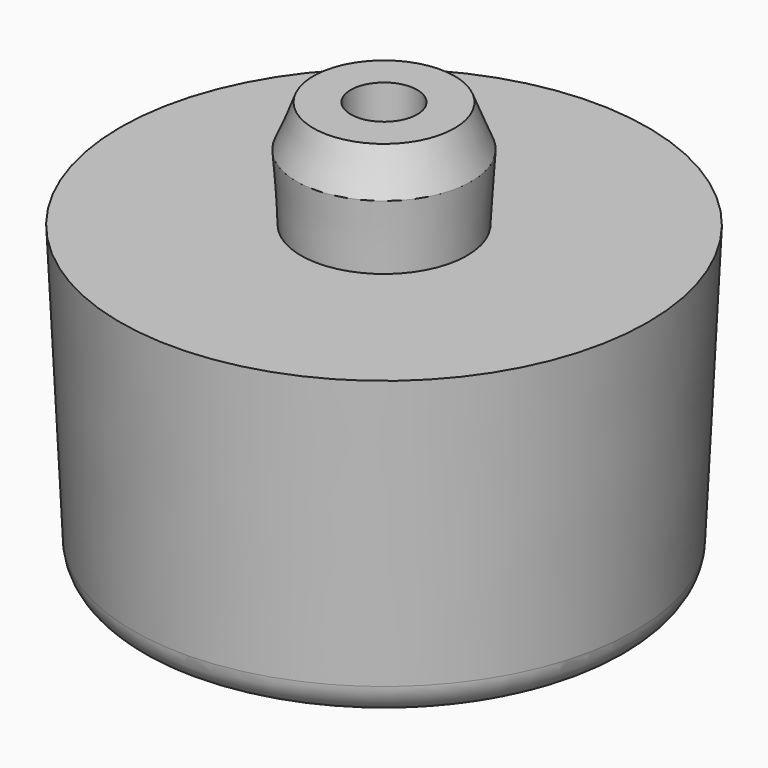
from build123d import *

# Parameters (mm, degrees)
F0_R      = 15
F2_R      = 15.875
F4_R      = 5
F6_R      = 5.25
F7_FACE_R = 5.25
F9_R      = 4.25
F11_R     = 2
F12_DEPTH = 25.0010001
F13_R     = 1.5
F15_R     = 2


with BuildPart() as f3:
    # F0 (on Top) → F3 section 0
    with BuildSketch(Plane.XY):
        Circle(F0_R)
    # F2 (on offset) → F3 section 1
    with BuildSketch(Plane.XY.offset(18.5)):
        Circle(F2_R)
    loft()

    # F4 (on face) → F7 section 0
    with BuildSketch(Plane.XY.offset(18.5)):
        Circle(F4_R)
    # F6 (on offset) → F7 section 1
    with BuildSketch(Plane.XY.offset(22.5)):
        Circle(F6_R)
    loft()

    # F7_face (on face) → F10 section 0
    with BuildSketch(Plane.XY.offset(22.5)):
        Circle(F7_FACE_R)
    # F9 (on offset) → F10 section 1
    with BuildSketch(Plane.XY.offset(25)):
        Circle(F9_R)
    loft()

    # F11 (on face) → F12 (cut, through all)
    with BuildSketch(Plane.XY.offset(25)):
        Circle(F11_R)
    extrude(amount=-F12_DEPTH, mode=Mode.SUBTRACT)

    # F13 (on Front) → F14 (revolve, cut)
    with BuildSketch(Plane.XZ):
        with Locations((-9.7052594647, 0)):
            Circle(F13_R)
    revolve(axis=Axis((0, 0, 7.5749068208), (0, 0, -1)), mode=Mode.SUBTRACT)

    # F15
    f15_edges = [f3.edges().sort_by_distance(p)[0] for p in [
        (-15, 0, 0),
    ]]
    fillet(f15_edges, radius=F15_R)


solid = f3.part
